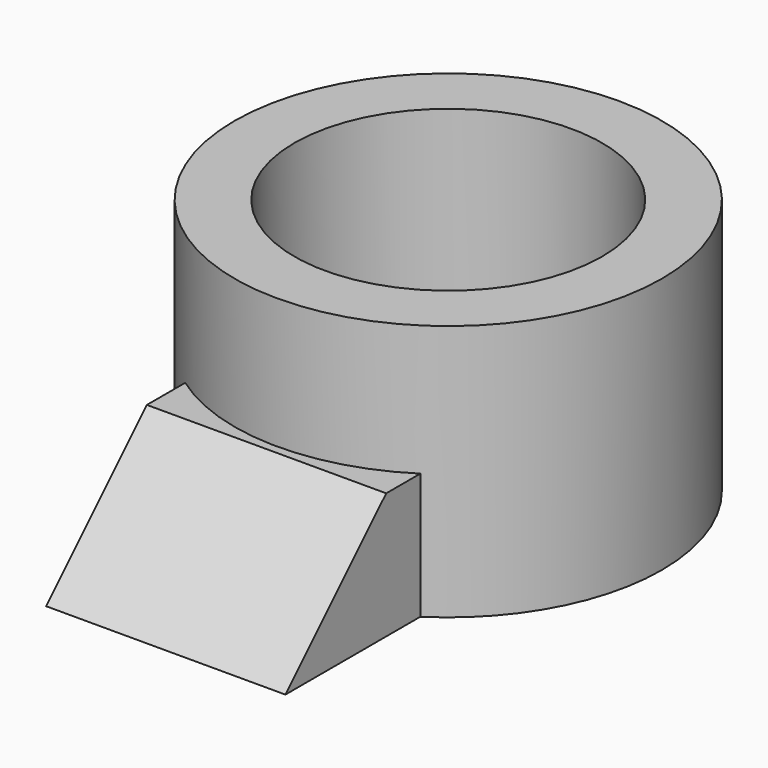
from build123d import *

# Parameters (mm, degrees)
F0_R        = 12.5
F1_DEPTH    = 7.5
F2_R        = 9
F3_DEPTH    = 25
F4_W        = 14
F4_H        = 7.3697703017
F5_DEPTH    = 23
F6_R        = 9
F7_DEPTH    = 25
F8_T1_DEPTH = 65.4336597593


# Not quite as in the source:
# - a fillet or chamfer that OpenCascade refuses, or shapes differently, is made with other operations: its cross-section is extruded or revolved along the edge and cut away or added


with BuildPart() as f1:
    # F0 (on Top) → F1 (new body, symmetric)
    with BuildSketch(Plane.XY):
        Circle(F0_R)
    extrude(amount=F1_DEPTH, both=True)

    # F2 (on face) → F3 (cut)
    with BuildSketch(Plane.XY.offset(7.5)):
        Circle(F2_R)
    extrude(amount=-F3_DEPTH, mode=Mode.SUBTRACT)

    # F4 (on Front) → F5 (join)
    with BuildSketch(Plane.XZ):
        with Locations((-0.2285402901, -3.8151148492)):
            Rectangle(F4_W, F4_H)
    extrude(amount=F5_DEPTH)

    # F6 (on face) → F7 (cut)
    with BuildSketch(Plane(origin=(0, 0, -7.5), x_dir=(1, 0, 0), z_dir=(0, 0, -1))):
        Circle(F6_R)
    extrude(amount=-F7_DEPTH, mode=Mode.SUBTRACT)

    # F8: chamfer of 10 on 1 edges, made by hand

    # F8_s2 → F8_t1 (cut)
    with BuildSketch(Plane.YZ.offset(-32.9453701698)):
        Polygon((-23, -10.1302296983), (-13, -0.1302296983), (-23, -0.1302296983), align=None)
    extrude(amount=F8_T1_DEPTH, mode=Mode.SUBTRACT)


solid = f1.part
